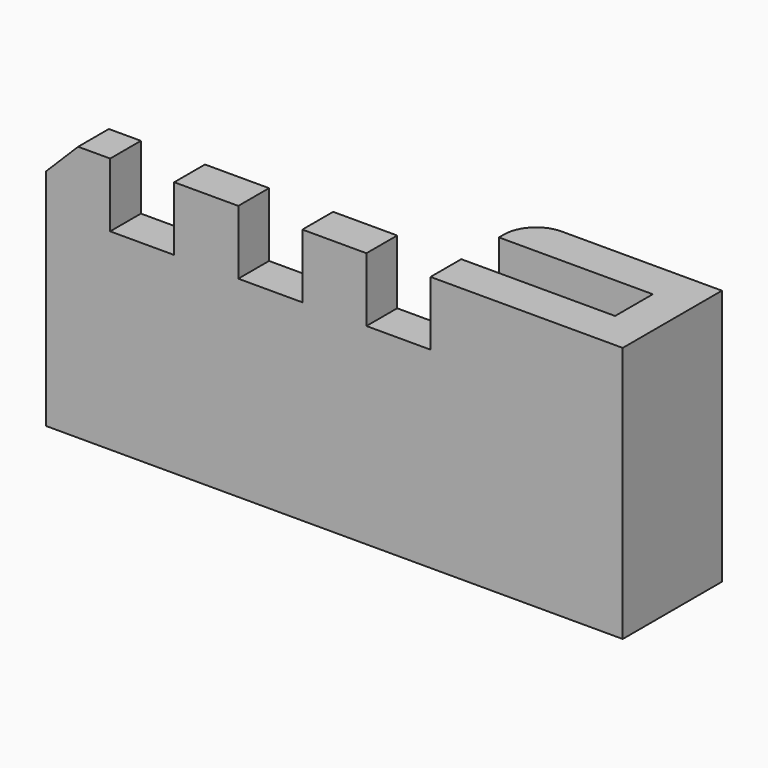
from build123d import *

# Parameters (mm, degrees)
F1_DEPTH = 20
F2_W     = 5
F2_H     = 5
F3_DEPTH = 14.204988947
F4_SIZE  = 2.5
F5_R     = 2.5


# Not quite as in the source:
# - a feature names something its author has since deleted; it is built from what else it names


with BuildPart() as f1:
    # F0 (on Top) → F1 (new body)
    with BuildSketch(Plane.XY):
        Polygon((0, -14.203988947), (0, -4.5276075453), (-15, -4.5276075453), (-15, -7.5276075453), (-2.9953992926, -7.5276075453), (-2.9953992926, -11.203988947), (-45, -11.203988947), (-45, -14.203988947), align=None)
    extrude(amount=F1_DEPTH)

    # F2 (on Front) → F3 (cut, through all)
    with BuildSketch(Plane.XZ):
        Polygon((-15, 17.4460405111), (-15, 20), (-20, 20), (-20, 15), (-15, 15), align=None)
        with Locations((-27.5, 17.5)):
            Rectangle(F2_W, F2_H)
        with Locations((-37.5, 17.5)):
            Rectangle(F2_W, F2_H)
    extrude(amount=F3_DEPTH, mode=Mode.SUBTRACT)

    # F4
    f4_edges = [f1.edges().sort_by_distance(p)[0] for p in [
        (-45, -12.703989, 20),
    ]]
    chamfer(f4_edges, length=F4_SIZE)

    # F5
    f5_edges = [f1.edges().sort_by_distance(p)[0] for p in [
        (-15, -4.527608, 10),
    ]]
    fillet(f5_edges, radius=F5_R)


solid = f1.part
